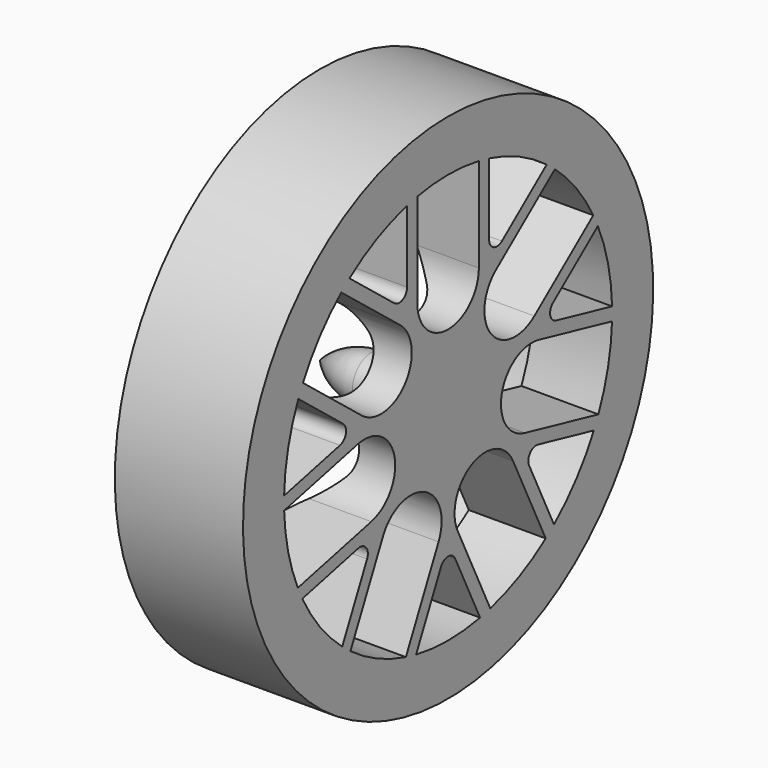
from build123d import *
from build123d import SkipClean  # not in build123d's __all__

# Parameters (mm, degrees)
F3_DEPTH      = 10
F3_DEPTH_BACK = 10
F5_DEPTH      = 0.1946
F5_DEPTH_BACK = 1


with BuildPart() as f1:
    # F0 (on Front) → F1 (revolve)
    with BuildSketch(Plane.XZ):
        with BuildLine():
            Line((2, 10), (0, 10))
            Line((0, 10), (-3, 10))
            Line((-3, 10), (-3, 9.5))
            Line((-3, 9.5), (-1, 9.5))
            Line((-1, 9.5), (-1, 6.8274233814))
            ThreePointArc((-1, 6.8274233814), (-0.6744935437, 4.9999678627), (0.2619870771, 3.397297537))
            ThreePointArc((0.2619870771, 3.397297537), (0.5273995547, 2.9430770304), (0.6196529053, 2.425149071))
            Line((0.6196529053, 2.425149071), (0.6196529053, 1.580287341))
            ThreePointArc((0.6196529053, 1.580287341), (0.330953643, 1.1028671143), (-0.1945994736, 0.9155938953))
            Line((-0.1945994736, 0.9155938953), (-1, 0.9155938953))
            ThreePointArc((-1, 0.9155938953), (-2.0998081857, 0.675815408), (-3, 0))
            Line((-3, 0), (2, 0))
            Line((2, 0), (2, 10))
        make_face()
    revolve(axis=Axis((0.9614995215, 0, 0), (1, 0, 0)))

    # F2 (on Right) → F3 (cut, two sides)
    with BuildSketch(Plane.YZ) as f3_sk:
        with BuildLine():
            Line((1.5, 4.1837804733), (1.5, 7.8581168228))
            ThreePointArc((1.5, 7.8581168228), (0, 8), (-1.5, 7.8581168228))
            Line((-1.5, 7.8581168228), (-1.5, 4.1837804733))
            ThreePointArc((-1.5, 4.1837804733), (0, 2.6837804733), (1.5, 4.1837804733))
        make_face()
        with BuildLine():
            ThreePointArc((-5.2084884222, 6.0722029245), (-6.2546518597, 4.9879184149), (-7.0789578277, 3.7267084771))
            Line((-7.0789578277, 3.7267084771), (-4.2062459926, 1.4357972346))
            ThreePointArc((-4.2062459926, 1.4357972346), (-2.0982640661, 1.6733097556), (-2.335776587, 3.781291682))
            Line((-2.335776587, 3.781291682), (-5.2084884222, 6.0722029245))
        make_face()
        with BuildLine():
            ThreePointArc((-7.9948788286, -0.2862036263), (-7.7994232975, -1.7801674717), (-7.3273160268, -3.2109873628))
            Line((-7.3273160268, -3.2109873628), (-3.745102961, -2.3933706067))
            ThreePointArc((-3.745102961, -2.3933706067), (-2.6164924936, -0.5971973375), (-4.4126657628, 0.5314131299))
            Line((-4.4126657628, 0.5314131299), (-7.9948788286, -0.2862036263))
        make_face()
        with BuildLine():
            ThreePointArc((-4.7609624113, -6.429093009), (-3.4710699129, -7.2077509432), (-2.0580558076, -7.7307442263))
            Line((-2.0580558076, -7.7307442263), (-0.4638210136, -4.4202815653))
            ThreePointArc((-0.4638210136, -4.4202815653), (-1.1644487067, -2.4180026548), (-3.1667276173, -3.1186303479))
            Line((-3.1667276173, -3.1186303479), (-4.7609624113, -6.429093009))
        make_face()
        with BuildLine():
            ThreePointArc((2.0580558076, -7.7307442263), (3.4710699129, -7.2077509432), (4.7609624113, -6.429093009))
            Line((4.7609624113, -6.429093009), (3.1667276173, -3.1186303479))
            ThreePointArc((3.1667276173, -3.1186303479), (1.1644487067, -2.4180026548), (0.4638210136, -4.4202815653))
            Line((0.4638210136, -4.4202815653), (2.0580558076, -7.7307442263))
        make_face()
        with BuildLine():
            ThreePointArc((7.3273160268, -3.2109873628), (7.7994232975, -1.7801674717), (7.9948788286, -0.2862036263))
            Line((7.9948788286, -0.2862036263), (4.4126657628, 0.5314131299))
            ThreePointArc((4.4126657628, 0.5314131299), (2.6164924936, -0.5971973375), (3.745102961, -2.3933706067))
            Line((3.745102961, -2.3933706067), (7.3273160268, -3.2109873628))
        make_face()
        with BuildLine():
            ThreePointArc((7.0789578277, 3.7267084771), (6.2546518597, 4.9879184149), (5.2084884222, 6.0722029245))
            Line((5.2084884222, 6.0722029245), (2.335776587, 3.781291682))
            ThreePointArc((2.335776587, 3.781291682), (2.0982640661, 1.6733097556), (4.2062459926, 1.4357972346))
            Line((4.2062459926, 1.4357972346), (7.0789578277, 3.7267084771))
        make_face()
        with BuildLine():
            Line((-2, 4.9505361331), (-2, 7.7459666924))
            ThreePointArc((-2, 7.7459666924), (-3.4710699129, 7.2077509432), (-4.8090610186, 6.3931942032))
            Line((-4.8090610186, 6.3931942032), (-2.6235054002, 4.6502717577))
            ThreePointArc((-2.6235054002, 4.6502717577), (-2.2174183943, 4.6045167408), (-2, 4.9505361331))
        make_face()
        with BuildLine():
            Line((-5.1174646077, 1.5229458278), (-7.303020226, 3.2658682733))
            ThreePointArc((-7.303020226, 3.2658682733), (-7.7994232975, 1.7801674717), (-7.9968010032, 0.2262160816))
            Line((-7.9968010032, 0.2262160816), (-5.2714577243, 0.8482579004))
            ThreePointArc((-5.2714577243, 0.8482579004), (-4.9824939048, 1.13722172), (-5.1174646077, 1.5229458278))
        make_face()
        with BuildLine():
            Line((-4.3813739885, -3.0514537483), (-7.1067172674, -3.6734955672))
            ThreePointArc((-7.1067172674, -3.6734955672), (-6.2546518597, -4.9879184149), (-5.1627867274, -6.1111073634))
            Line((-5.1627867274, -6.1111073634), (-3.9498948639, -3.5925114571))
            ThreePointArc((-3.9498948639, -3.5925114571), (-3.9956498807, -3.1864244511), (-4.3813739885, -3.0514537483))
        make_face()
        with BuildLine():
            Line((-0.3460193923, -5.3280464136), (-1.5589112558, -7.8466423199))
            ThreePointArc((-1.5589112558, -7.8466423199), (0, -8), (1.5589112558, -7.8466423199))
            Line((1.5589112558, -7.8466423199), (0.3460193923, -5.3280464136))
            ThreePointArc((0.3460193923, -5.3280464136), (0, -5.1106280193), (-0.3460193923, -5.3280464136))
        make_face()
        with BuildLine():
            Line((3.9498948639, -3.5925114571), (5.1627867274, -6.1111073634))
            ThreePointArc((5.1627867274, -6.1111073634), (6.2546518597, -4.9879184149), (7.1067172674, -3.6734955672))
            Line((7.1067172674, -3.6734955672), (4.3813739885, -3.0514537483))
            ThreePointArc((4.3813739885, -3.0514537483), (3.9956498807, -3.1864244511), (3.9498948639, -3.5925114571))
        make_face()
        with BuildLine():
            Line((5.2714577243, 0.8482579004), (7.9968010032, 0.2262160816))
            ThreePointArc((7.9968010032, 0.2262160816), (7.7994232975, 1.7801674717), (7.303020226, 3.2658682733))
            Line((7.303020226, 3.2658682733), (5.1174646077, 1.5229458278))
            ThreePointArc((5.1174646077, 1.5229458278), (4.9824939048, 1.13722172), (5.2714577243, 0.8482579004))
        make_face()
        with BuildLine():
            Line((2.6235054002, 4.6502717577), (4.8090610186, 6.3931942032))
            ThreePointArc((4.8090610186, 6.3931942032), (3.4710699129, 7.2077509432), (2, 7.7459666924))
            Line((2, 7.7459666924), (2, 4.9505361331))
            ThreePointArc((2, 4.9505361331), (2.2174183943, 4.6045167408), (2.6235054002, 4.6502717577))
        make_face()
    extrude(amount=-F3_DEPTH, mode=Mode.SUBTRACT)
    extrude(f3_sk.sketch, amount=F3_DEPTH_BACK, mode=Mode.SUBTRACT)

    # F4 (on Right) → F5 (cut, two sides)
    with BuildSketch(Plane.YZ) as f5_sk:
        with BuildLine():
            ThreePointArc((0.4100744534, 1.5261543247), (0, 1.580287341), (-0.4100744534, 1.5261543247))
            Line((-0.4100744534, 1.5261543247), (-0.2380390581, 0.8841094886))
            ThreePointArc((-0.2380390581, 0.8841094886), (0, 0.9155938953), (0.2380390581, 0.8841094886))
            Line((0.2380390581, 0.8841094886), (0.4100744534, 1.5261543247))
        make_face()
        with BuildLine():
            ThreePointArc((-0.7934788469, 0.4568407826), (-0.6474226522, 0.6474226522), (-0.4568407826, 0.7934788469))
            Line((-0.4568407826, 0.7934788469), (-0.7891876453, 1.3691204989))
            ThreePointArc((-0.7891876453, 1.3691204989), (-1.117431895, 1.117431895), (-1.3691204989, 0.7891876453))
            Line((-1.3691204989, 0.7891876453), (-0.7934788469, 0.4568407826))
        make_face()
        with BuildLine():
            ThreePointArc((-0.8841094886, -0.2380390581), (-0.9155938953, 0), (-0.8841094886, 0.2380390581))
            Line((-0.8841094886, 0.2380390581), (-1.5261543247, 0.4100744534))
            ThreePointArc((-1.5261543247, 0.4100744534), (-1.580287341, 0), (-1.5261543247, -0.4100744534))
            Line((-1.5261543247, -0.4100744534), (-0.8841094886, -0.2380390581))
        make_face()
        with BuildLine():
            ThreePointArc((-0.4568407826, -0.7934788469), (-0.6474226522, -0.6474226522), (-0.7934788469, -0.4568407826))
            Line((-0.7934788469, -0.4568407826), (-1.3691204989, -0.7891876453))
            ThreePointArc((-1.3691204989, -0.7891876453), (-1.117431895, -1.117431895), (-0.7891876453, -1.3691204989))
            Line((-0.7891876453, -1.3691204989), (-0.4568407826, -0.7934788469))
        make_face()
        with BuildLine():
            ThreePointArc((0.2380390581, -0.8841094886), (0, -0.9155938953), (-0.2380390581, -0.8841094886))
            Line((-0.2380390581, -0.8841094886), (-0.4100744534, -1.5261543247))
            ThreePointArc((-0.4100744534, -1.5261543247), (0, -1.580287341), (0.4100744534, -1.5261543247))
            Line((0.4100744534, -1.5261543247), (0.2380390581, -0.8841094886))
        make_face()
        with BuildLine():
            ThreePointArc((0.7934788469, -0.4568407826), (0.6474226522, -0.6474226522), (0.4568407826, -0.7934788469))
            Line((0.4568407826, -0.7934788469), (0.7891876453, -1.3691204989))
            ThreePointArc((0.7891876453, -1.3691204989), (1.117431895, -1.117431895), (1.3691204989, -0.7891876453))
            Line((1.3691204989, -0.7891876453), (0.7934788469, -0.4568407826))
        make_face()
        with BuildLine():
            ThreePointArc((0.8841094886, 0.2380390581), (0.9155938953, 0), (0.8841094886, -0.2380390581))
            Line((0.8841094886, -0.2380390581), (1.5261543247, -0.4100744534))
            ThreePointArc((1.5261543247, -0.4100744534), (1.580287341, 0), (1.5261543247, 0.4100744534))
            Line((1.5261543247, 0.4100744534), (0.8841094886, 0.2380390581))
        make_face()
        with BuildLine():
            ThreePointArc((0.4568407826, 0.7934788469), (0.6474226522, 0.6474226522), (0.7934788469, 0.4568407826))
            Line((0.7934788469, 0.4568407826), (1.3691204989, 0.7891876453))
            ThreePointArc((1.3691204989, 0.7891876453), (1.117431895, 1.117431895), (0.7891876453, 1.3691204989))
            Line((0.7891876453, 1.3691204989), (0.4568407826, 0.7934788469))
        make_face()
    with SkipClean():  # cleaning this boolean's faces spoils the solid; the shape is the same uncleaned
        extrude(amount=-F5_DEPTH, mode=Mode.SUBTRACT)
        extrude(f5_sk.sketch, amount=F5_DEPTH_BACK, mode=Mode.SUBTRACT)


solid = f1.part
